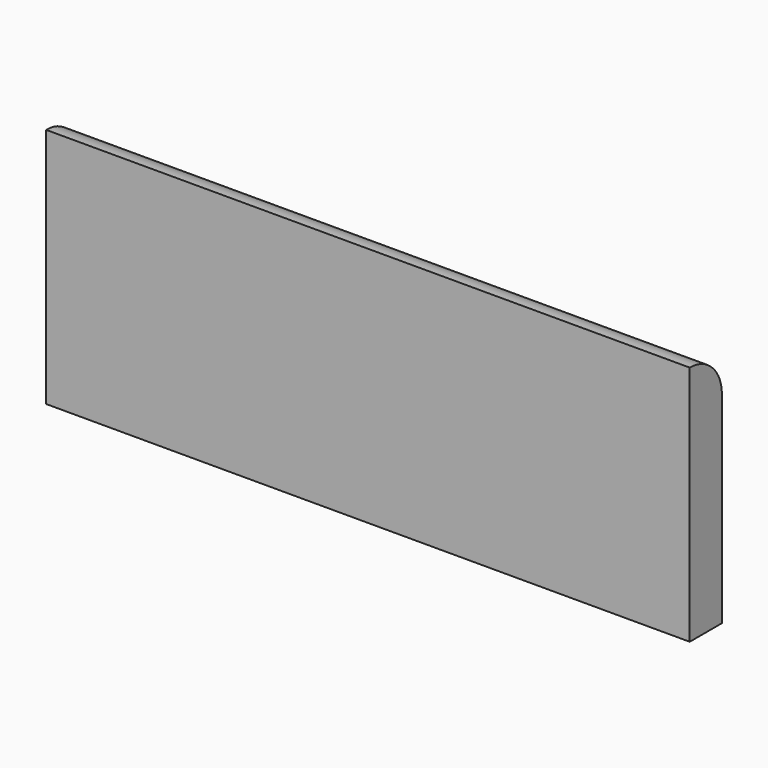
from build123d import *

# Parameters (mm, degrees)
F0_W     = 203.2
F0_H     = 76.2
F1_DEPTH = 12.7
F2_R     = 12.69999


# Not quite as in the source:
# - a fillet or chamfer is up to 0.001 mm smaller than in the source, because OpenCascade refuses the exact size


with BuildPart() as f1:
    # F0 (on Front) → F1 (new body)
    with BuildSketch(Plane.XZ):
        Rectangle(F0_W, F0_H)
    extrude(amount=F1_DEPTH)

    # F2 (radius 12.7 in the source; OpenCascade refuses exactly that, so slightly less here)
    f2_edges = [f1.edges().sort_by_distance(p)[0] for p in [
        (0, 0, 38.1),
    ]]
    fillet(f2_edges, radius=F2_R)


solid = f1.part
